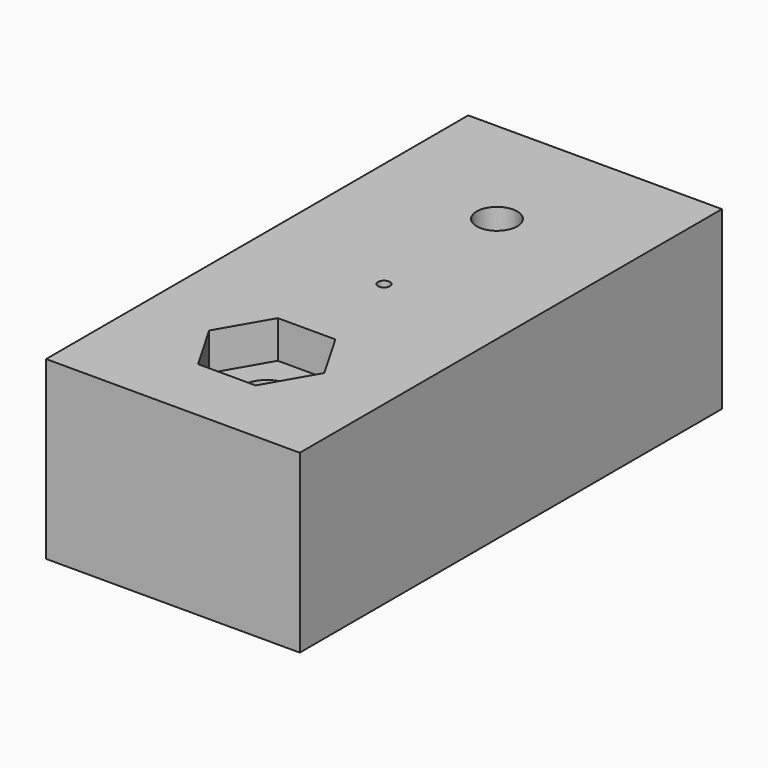
from build123d import *

# Parameters (mm, degrees)
F0_W     = 21.6265451163
F0_H     = 44.9824891984
F0_R     = 0.5
F0_R_2   = 1.7272
F0_R_3   = 2.085
F1_DEPTH = 15
F2_DEPTH = 3.2


# Not quite as in the source:
# - a feature names something its author has since deleted; it is built from what else it names


with BuildPart() as f1:
    # F0 (on Top) → F1 (new body)
    with BuildSketch(Plane.XY):
        Rectangle(F0_W, F0_H)
        Polygon((-4.9074772881, -12.4994842336), (-2.4537386441, -8.2494842336), (2.4537386441, -8.2494842336), (4.9074772881, -12.4994842336), (2.4537386441, -16.7494842336), (-2.4537386441, -16.7494842336), align=None, mode=Mode.SUBTRACT)
        Circle(F0_R, mode=Mode.SUBTRACT)
        with Locations((0, 12.0378434658)):
            Circle(F0_R_2, mode=Mode.SUBTRACT)
        Polygon((2.4537386441, -8.2494842336), (-2.4537386441, -8.2494842336), (-4.9074772881, -12.4994842336), (-2.4537386441, -16.7494842336), (2.4537386441, -16.7494842336), (4.9074772881, -12.4994842336), align=None)
        with Locations((0, -12.4994842336)):
            Circle(F0_R_3, mode=Mode.SUBTRACT)
    extrude(amount=-F1_DEPTH)

    # F0 (on Top) → F2 (cut)
    with BuildSketch(Plane.XY):
        Polygon((2.4537386441, -8.2494842336), (-2.4537386441, -8.2494842336), (-4.9074772881, -12.4994842336), (-2.4537386441, -16.7494842336), (2.4537386441, -16.7494842336), (4.9074772881, -12.4994842336), align=None)
        with Locations((0, -12.4994842336)):
            Circle(F0_R_3, mode=Mode.SUBTRACT)
    extrude(amount=-F2_DEPTH, mode=Mode.SUBTRACT)


solid = f1.part
